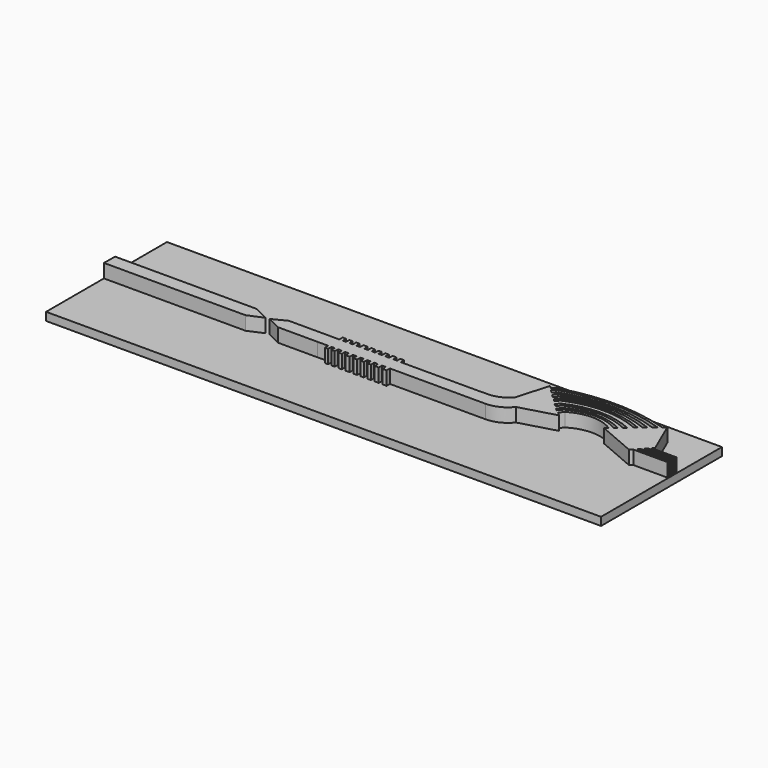
from build123d import *

# Parameters (mm, degrees)
F0_W     = 505.468076095
F0_H     = 137.6467421651
F1_DEPTH = 7.366
F3_DEPTH = 12.446


# Not quite as in the source:
# - a feature names something its author has since deleted; it is built from what else it names


with BuildPart() as f1:
    # F0 (on Top) → F1 (new body)
    with BuildSketch(Plane.XY):
        with Locations((232.2135167196, 0.7967613637)):
            Rectangle(F0_W, F0_H)
    extrude(amount=F1_DEPTH)

    # F2 (on face) → F3 (join)
    with BuildSketch(Plane.XY.offset(7.366)):
        with BuildLine():
            Line((183.8642209768, 14.1799058765), (183.8642209768, 10.2725932375))
            Line((183.8642209768, 10.2725932375), (181.7528605461, 10.280970484))
            Line((181.7528605461, 10.280970484), (174.2617040873, 10.3483377025))
            Line((174.2617040873, 10.3483377025), (137.7773582935, 10.3483377025))
            Line((137.7773582935, 10.3483377025), (125.377446413, 4.0150946006))
            Line((125.377446413, 4.0150946006), (138.0158215761, -2.1848597098))
            Line((138.0158215761, -2.1848597098), (174.0232408047, -2.1848597098))
            Line((174.0232408047, -2.1848597098), (181.7289143801, -2.1529737648))
            Line((181.7289143801, -2.1529737648), (183.6102157831, -2.1509330043))
            Line((183.6102157831, -2.1509330043), (183.5907548666, -5.8423327282))
            Line((183.5907548666, -5.8423327282), (186.6615414619, -5.8423327282))
            Line((186.6615414619, -5.8423327282), (186.6615414619, -2.0806165412))
            Line((186.6615414619, -2.0806165412), (189.655572176, -2.0806165412))
            Line((189.655572176, -2.0806165412), (189.655572176, -5.8423327282))
            Line((189.655572176, -5.8423327282), (192.6495879889, -5.8423327282))
            Line((192.6495879889, -5.8423327282), (192.6495879889, -2.0806165412))
            Line((192.6495879889, -2.0806165412), (195.8739161491, -2.0806165412))
            Line((195.8739161491, -2.0806165412), (195.8739161491, -5.8423327282))
            Line((195.8739161491, -5.8423327282), (199.0982443094, -5.8423327282))
            Line((199.0982443094, -5.8423327282), (199.0982443094, -2.0806165412))
            Line((199.0982443094, -2.0806165412), (202.4761140347, -2.0806165412))
            Line((202.4761140347, -2.0806165412), (202.4761140347, -5.8423327282))
            Line((202.4761140347, -5.8423327282), (206.2378227711, -5.8423327282))
            Line((206.2378227711, -5.8423327282), (206.2378227711, -2.0806165412))
            Line((206.2378227711, -2.0806165412), (209.6156924963, -2.0806165412))
            Line((209.6156924963, -2.0806165412), (209.6156924963, -5.8423327282))
            Line((209.6156924963, -5.8423327282), (213.1471037865, -5.8423327282))
            Line((213.1471037865, -5.8423327282), (213.1471037865, -2.0806165412))
            Line((213.1471037865, -2.0806165412), (216.1411345005, -2.0806165412))
            Line((216.1411345005, -2.0806165412), (216.1411345005, -5.8423327282))
            Line((216.1411345005, -5.8423327282), (219.1351503134, -5.8423327282))
            Line((219.1351503134, -5.8423327282), (219.1351503134, -2.0806165412))
            Line((219.1351503134, -2.0806165412), (222.3594784737, -2.0806165412))
            Line((222.3594784737, -2.0806165412), (222.3594784737, -5.8423327282))
            Line((222.3594784737, -5.8423327282), (225.5838066339, -5.8423327282))
            Line((225.5838066339, -5.8423327282), (225.5838066339, -2.0806165412))
            Line((225.5838066339, -2.0806165412), (228.9616763592, -2.0806165412))
            Line((228.9616763592, -2.0806165412), (228.9616763592, -5.8423327282))
            Line((228.9616763592, -5.8423327282), (232.7233850956, -5.8423327282))
            Line((232.7233850956, -5.8423327282), (232.7233850956, -2.0806165412))
            Line((232.7233850956, -2.0806165412), (236.1012548208, -2.0806165412))
            Line((236.1012548208, -2.0806165412), (236.1012548208, -5.8423327282))
            Line((236.1012548208, -5.8423327282), (239.886666111, -5.8423327282))
            Line((239.886666111, -5.8423327282), (239.886666111, -2.0361929703))
            Line((239.886666111, -2.0361929703), (308.7113499641, -2.0361929703))
            Line((308.7113499641, -2.0361929703), (327.0893990993, -2.0361929703))
            ThreePointArc((327.0893990993, -2.0361929703), (338.0716042416, 0.4904142901), (346.8455672264, 7.5621996075))
            Line((346.8455672264, 7.5621996075), (379.0387098504, 16.6834991227))
            Line((379.0387098504, 16.6834991227), (375.7017479006, 19.6033408288))
            Line((375.7017479006, 19.6033408288), (379.0387098504, 23.4170116286))
            ThreePointArc((379.0387098504, 23.4170116286), (399.0077273508, 29.2230595274), (418.9767448512, 23.4170116286))
            Line((418.9767448512, 23.4170116286), (416.3737297058, 21.2878081948))
            Line((416.3737297058, 21.2878081948), (450.9352743626, 6.4515918493))
            Line((450.9352743626, 6.4515918493), (453.2975118055, 8.5896141827))
            Line((453.2975118055, 8.5896141827), (484.4302535057, 8.5896141827))
            Line((484.4302535057, 8.5896141827), (484.4302535057, 10.8214179054))
            Line((484.4302535057, 10.8214179054), (454.9943455488, 10.8214179054))
            Line((454.9943455488, 10.8214179054), (457.0494721473, 12.6347579062))
            Line((457.0494721473, 12.6347579062), (484.4302535057, 12.6347579062))
            Line((484.4302535057, 12.6347579062), (484.4302535057, 14.448097907))
            Line((484.4302535057, 14.448097907), (457.9519460917, 14.448097907))
            Line((457.9519460917, 14.448097907), (460.04427444, 16.5404137224))
            Line((460.04427444, 16.5404137224), (484.4302535057, 16.5404137224))
            Line((484.4302535057, 16.5404137224), (484.4302535057, 18.3537546545))
            Line((484.4302535057, 18.3537546545), (461.2901464378, 18.3537546545))
            Line((461.2901464378, 18.3537546545), (463.6734724045, 20.1696325094))
            Line((463.6734724045, 20.1696325094), (450.5897462368, 50.3342226148))
            Line((450.5897462368, 50.3342226148), (447.8478631112, 48.0109341443))
            ThreePointArc((447.8478631112, 48.0109341443), (399.0077273508, 55.560682533), (350.1675915904, 48.0109341443))
            Line((350.1675915904, 48.0109341443), (348.1977880001, 45.759730041))
            Line((348.1977880001, 45.759730041), (345.6249833107, 48.0109341443))
            Line((345.6249833107, 48.0109341443), (336.9521223247, 17.9653423708))
            ThreePointArc((336.9521223247, 17.9653423708), (327.6334286446, 12.1000348485), (316.7435458205, 10.4720494957))
            Line((316.7435458205, 10.4720494957), (309.5143437386, 10.3298625909))
            Line((309.5143437386, 10.3298625909), (239.8866713047, 10.3298625909))
            Line((239.8866713047, 10.3298625909), (239.8866713047, 14.1799058765))
            Line((239.8866713047, 14.1799058765), (236.3552600145, 14.1799058765))
            Line((236.3552600145, 14.1799058765), (236.3552600145, 10.4181896895))
            Line((236.3552600145, 10.4181896895), (232.9773902893, 10.4181896895))
            Line((232.9773902893, 10.4181896895), (232.9773902893, 14.1799058765))
            Line((232.9773902893, 14.1799058765), (229.2156815529, 14.1799058765))
            Line((229.2156815529, 14.1799058765), (229.2156815529, 10.4181896895))
            Line((229.2156815529, 10.4181896895), (225.8378118277, 10.4181896895))
            Line((225.8378118277, 10.4181896895), (225.8378118277, 14.1799058765))
            Line((225.8378118277, 14.1799058765), (222.6134836674, 14.1799058765))
            Line((222.6134836674, 14.1799058765), (222.6134836674, 10.4181896895))
            Line((222.6134836674, 10.4181896895), (219.3891555071, 10.4181896895))
            Line((219.3891555071, 10.4181896895), (219.3891555071, 14.1799058765))
            Line((219.3891555071, 14.1799058765), (216.3951396942, 14.1799058765))
            Line((216.3951396942, 14.1799058765), (216.3951396942, 10.4181896895))
            Line((216.3951396942, 10.4181896895), (213.4011089802, 10.4181896895))
            Line((213.4011089802, 10.4181896895), (213.4011089802, 14.1799058765))
            Line((213.4011089802, 14.1799058765), (209.86969769, 14.1799058765))
            Line((209.86969769, 14.1799058765), (209.86969769, 10.4181896895))
            Line((209.86969769, 10.4181896895), (206.4918279648, 10.4181896895))
            Line((206.4918279648, 10.4181896895), (206.4918279648, 14.1799058765))
            Line((206.4918279648, 14.1799058765), (202.7301192284, 14.1799058765))
            Line((202.7301192284, 14.1799058765), (202.7301192284, 10.4181896895))
            Line((202.7301192284, 10.4181896895), (199.3522495031, 10.4181896895))
            Line((199.3522495031, 10.4181896895), (199.3522495031, 14.1799058765))
            Line((199.3522495031, 14.1799058765), (196.1279213428, 14.1799058765))
            Line((196.1279213428, 14.1799058765), (196.1279213428, 10.4181896895))
            Line((196.1279213428, 10.4181896895), (192.9035931826, 10.4181896895))
            Line((192.9035931826, 10.4181896895), (192.9035931826, 14.1799058765))
            Line((192.9035931826, 14.1799058765), (189.9095773697, 14.1799058765))
            Line((189.9095773697, 14.1799058765), (189.9095773697, 10.4181896895))
            Line((189.9095773697, 10.4181896895), (186.9155466557, 10.4181896895))
            Line((186.9155466557, 10.4181896895), (186.9155466557, 14.1799058765))
            Line((186.9155466557, 14.1799058765), (183.8642209768, 14.1799058765))
        make_face()
        with BuildLine():
            Line((370.6372472565, 23.5322912479), (374.053896924, 27.4370337251))
            ThreePointArc((374.053896924, 27.4370337251), (399.0077273508, 33.7810246324), (423.9615577776, 27.4370337251))
            Line((423.9615577776, 27.4370337251), (421.708929064, 25.8076728149))
            ThreePointArc((421.708929064, 25.8076728149), (399.0077273508, 31.9265013842), (376.3065256376, 25.8076728149))
            Line((376.3065256376, 25.8076728149), (372.7205432622, 21.7094072429))
            Line((372.7205432622, 21.7094072429), (370.6372472565, 23.5322912479))
        make_face(mode=Mode.SUBTRACT)
        with BuildLine():
            Line((365.6382056992, 28.3170708711), (368.6322219076, 31.7388036808))
            ThreePointArc((368.6322219076, 31.7388036808), (399.0077273508, 38.526410097), (429.383232794, 31.7388036808))
            Line((429.383232794, 31.7388036808), (426.7392740049, 29.867535424))
            ThreePointArc((426.7392740049, 29.867535424), (399.0077273508, 36.4081558373), (371.2761806967, 29.867535424))
            Line((371.2761806967, 29.867535424), (368.0630232644, 26.1953555015))
            Line((368.0630232644, 26.1953555015), (365.6382056992, 28.3170708711))
        make_face(mode=Mode.SUBTRACT)
        with BuildLine():
            Line((360.4813304683, 33.5443242144), (363.4392711441, 36.9248278439))
            ThreePointArc((363.4392711441, 36.9248278439), (399.0077273508, 44.2750490819), (434.5761835575, 36.9248278439))
            Line((434.5761835575, 36.9248278439), (432.3772490025, 35.0923612714))
            ThreePointArc((432.3772490025, 35.0923612714), (399.0077273508, 42.2705737087), (365.6382056992, 35.0923612714))
            Line((365.6382056992, 35.0923612714), (362.6348697567, 31.6599773371))
            Line((362.6348697567, 31.6599773371), (360.4813304683, 33.5443242144))
        make_face(mode=Mode.SUBTRACT)
        with BuildLine():
            Line((355.3299033536, 38.152305195), (358.0891265806, 41.3057031687))
            ThreePointArc((358.0891265806, 41.3057031687), (399.0077273508, 48.9346794019), (439.926328121, 41.3057031687))
            Line((439.926328121, 41.3057031687), (436.997769417, 39.1854137116))
            ThreePointArc((436.997769417, 39.1854137116), (399.0077273508, 46.6356083993), (361.0176852847, 39.1854137116))
            Line((361.0176852847, 39.1854137116), (358.0393189878, 35.7815665152))
            Line((358.0393189878, 35.7815665152), (355.3299033536, 38.152305195))
        make_face(mode=Mode.SUBTRACT)
        with BuildLine():
            Line((350.1675915904, 43.2099050709), (352.5468626356, 45.9290719797))
            ThreePointArc((352.5468626356, 45.9290719797), (399.0077273508, 53.6790820799), (445.468592066, 45.9290719797))
            Line((445.468592066, 45.9290719797), (442.4422114296, 43.5071010637))
            ThreePointArc((442.4422114296, 43.5071010637), (399.0077273508, 51.1039718638), (355.573243272, 43.5071010637))
            Line((355.573243272, 43.5071010637), (353.0819166526, 40.6598706415))
            Line((353.0819166526, 40.6598706415), (350.1675915904, 43.2099050709))
        make_face(mode=Mode.SUBTRACT)
        Polygon((108.4468066692, -2.1848597098), (122.0492497087, 3.6468699109), (108.5446923971, 10.3483377025), (-20.3237645328, 10.3483377025), (-20.5205213279, -2.1848597098), align=None)
    extrude(amount=F3_DEPTH)


solid = f1.part
